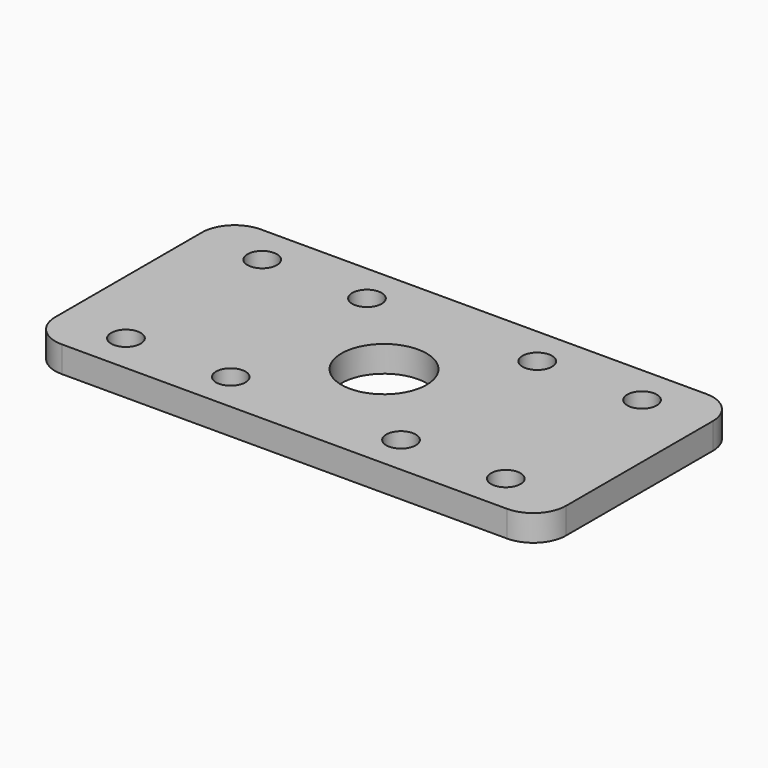
from build123d import *

# Parameters (mm, degrees)
F0_W     = 78
F0_H     = 38
F0_R     = 2.25
F0_R_2   = 6.5
F1_DEPTH = 4
F2_R     = 5


# Not quite as in the source:
# - a feature names something its author has since deleted; it is built from what else it names


with BuildPart() as f1:
    # F0 (on Top) → F1 (new body)
    with BuildSketch(Plane.XY):
        Rectangle(F0_W, F0_H)
        with Locations((-29, -13)):
            Circle(F0_R, mode=Mode.SUBTRACT)
        with Locations((-13, -13)):
            Circle(F0_R, mode=Mode.SUBTRACT)
        with Locations((13, -13)):
            Circle(F0_R, mode=Mode.SUBTRACT)
        with Locations((29, -13)):
            Circle(F0_R, mode=Mode.SUBTRACT)
        with Locations((-29, 13)):
            Circle(F0_R, mode=Mode.SUBTRACT)
        with Locations((-13, 13)):
            Circle(F0_R, mode=Mode.SUBTRACT)
        Circle(F0_R_2, mode=Mode.SUBTRACT)
        with Locations((13, 13)):
            Circle(F0_R, mode=Mode.SUBTRACT)
        with Locations((29, 13)):
            Circle(F0_R, mode=Mode.SUBTRACT)
    extrude(amount=-F1_DEPTH)

    # F2
    f2_edges = [f1.edges().sort_by_distance(p)[0] for p in [
        (-39, -19, -2),
        (39, -19, -2),
        (39, 19, -2),
        (-39, 19, -2),
    ]]
    fillet(f2_edges, radius=F2_R)


solid = f1.part
